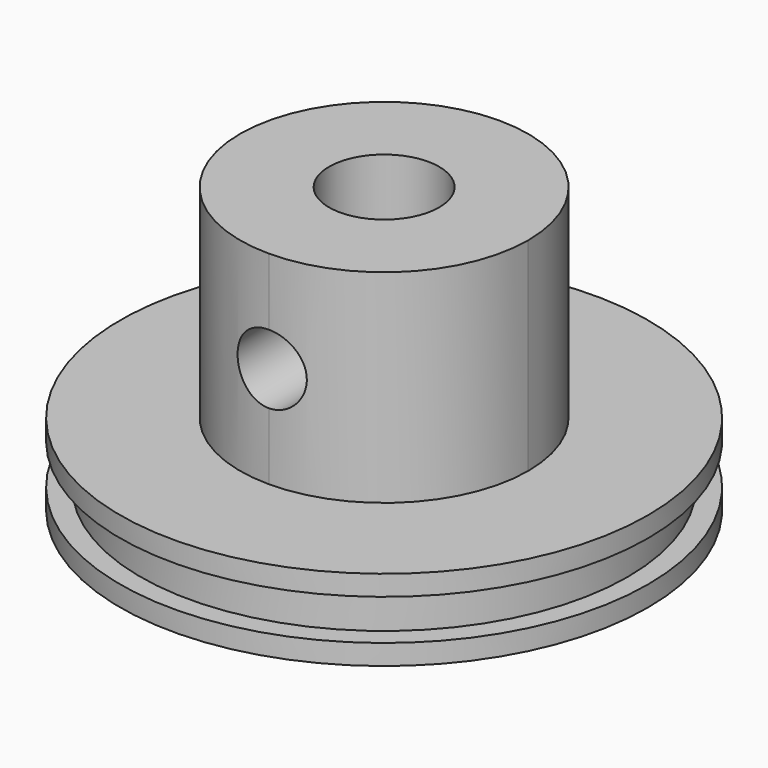
from build123d import *

# Parameters (mm, degrees)
F0_R        = 10.31875
F0_R_2      = 2.15265
F1_DEPTH    = 3.175
F2_W        = 11.2655872395
F2_H        = 11.2655872395
F2_R        = 2.15265
F3_DEPTH    = 7.9375
F4_R        = 1.35255
F5_REACH    = 19.7781327273
F6_T1_DEPTH = 22.01948225
F7_W        = 0.79375
F7_H        = 1.5875


# Not quite as in the source:
# - a fillet or chamfer that OpenCascade refuses, or shapes differently, is made with other operations: its cross-section is extruded or revolved along the edge and cut away or added


with BuildPart() as f1:
    # F0 (on Top) → F1 (new body)
    with BuildSketch(Plane.XY):
        Circle(F0_R)
        Circle(F0_R_2, mode=Mode.SUBTRACT)
    extrude(amount=F1_DEPTH)

    # F2 (on face) → F3 (join)
    with BuildSketch(Plane.XY.offset(3.175)):
        Rectangle(F2_W, F2_H)
        Circle(F2_R, mode=Mode.SUBTRACT)
    extrude(amount=F3_DEPTH)

    f5_end = f1.faces().sort_by_distance((-2.15265, 0, 5.55625))[0]
    # F4 (on face) → F5 (cut, up to a face of the model that its end follows)
    with BuildSketch(Plane.XZ.offset(5.6327936197)):
        with Locations((0, 7.14375)):
            Circle(F4_R)
    f5_long = extrude(amount=-F5_REACH, mode=Mode.PRIVATE)
    add(split(f5_long, bisect_by=f5_end, keep=Keep.ALL, mode=Mode.PRIVATE).solids().sort_by_distance((0, -5.6327936197, 7.14375))[0], mode=Mode.SUBTRACT)

    # F6: fillet of radius 5.6327929 on 4 edges, made by hand

    # F6_s2 → F6_t1 (cut)
    with BuildSketch(Plane.XY.offset(3.175)):
        with BuildLine():
            ThreePointArc((-5.6327936197, -7.197e-07), (-3.9829867763, -3.9829867763), (-7.197e-07, -5.6327936197))
            Line((-7.197e-07, -5.6327936197), (-5.6327936197, -5.6327936197))
            Line((-5.6327936197, -5.6327936197), (-5.6327936197, -7.197e-07))
        make_face()
        with BuildLine():
            ThreePointArc((7.197e-07, -5.6327936197), (3.9829867763, -3.9829867763), (5.6327936197, -7.197e-07))
            Line((5.6327936197, -7.197e-07), (5.6327936197, -5.6327936197))
            Line((5.6327936197, -5.6327936197), (7.197e-07, -5.6327936197))
        make_face()
        with BuildLine():
            ThreePointArc((7.197e-07, 5.6327936197), (3.9829867763, 3.9829867763), (5.6327936197, 7.197e-07))
            Line((5.6327936197, 7.197e-07), (5.6327936197, 5.6327936197))
            Line((5.6327936197, 5.6327936197), (7.197e-07, 5.6327936197))
        make_face()
        with BuildLine():
            ThreePointArc((-7.197e-07, 5.6327936197), (-3.9829867763, 3.9829867763), (-5.6327936197, 7.197e-07))
            Line((-5.6327936197, 7.197e-07), (-5.6327936197, 5.6327936197))
            Line((-5.6327936197, 5.6327936197), (-7.197e-07, 5.6327936197))
        make_face()
    extrude(amount=F6_T1_DEPTH, mode=Mode.SUBTRACT)

    # F7 (on Front) → F8 (revolve, cut)
    with BuildSketch(Plane.XZ):
        with Locations((9.921875, 1.5875)):
            Rectangle(F7_W, F7_H)
    revolve(axis=Axis((0, 0, 0), (0, 0, 1)), mode=Mode.SUBTRACT)


solid = f1.part
